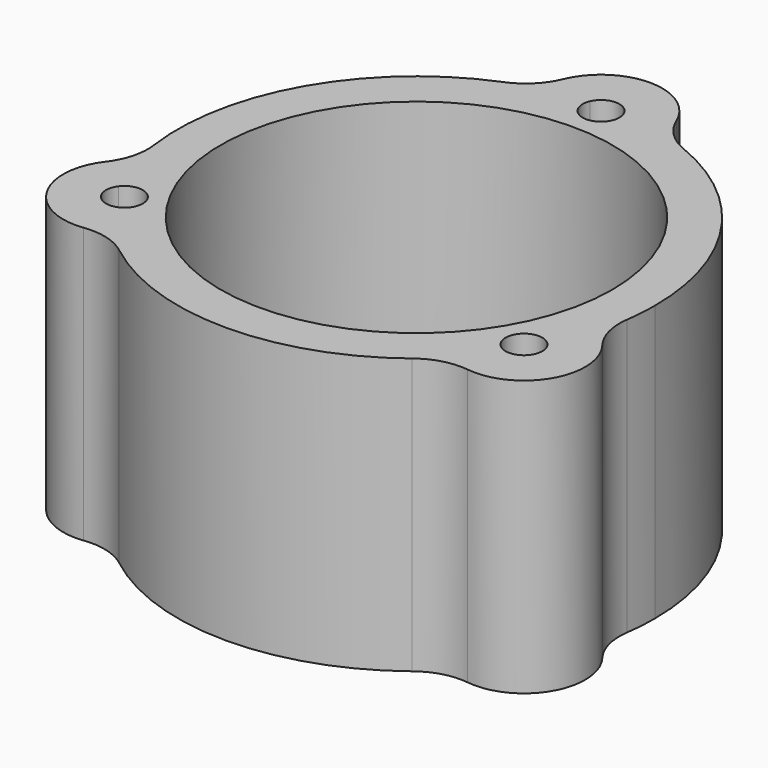
from build123d import *

# Parameters (mm, degrees)
F0_R     = 20.32
F1_DEPTH = 28.575
F2_R     = 6.35


with BuildPart() as f1:
    # F0 (on Top) → F1 (new body)
    with BuildSketch(Plane.XY):
        with BuildLine():
            ThreePointArc((23.9050999455, -6.4692674698), (24.5490837421, -3.2630832697), (24.765, 0))
            ThreePointArc((24.765, 0), (19.6285885254, 15.1004548773), (6.35, 23.9370575677))
            ThreePointArc((6.35, 23.9370575677), (4.0651088886, 24.4290833787), (1.7440091422, 24.703515076))
            ThreePointArc((1.7440091422, 24.703515076), (1.8643178935, 24.3286489263), (1.905, 23.9370575677))
            ThreePointArc((1.905, 23.9370575677), (-0.3915913586, 22.0727396742), (-1.7440091422, 24.703515076))
            ThreePointArc((-1.7440091422, 24.703515076), (-4.0651088886, 24.4290833787), (-6.35, 23.9370575677))
            ThreePointArc((-6.35, 23.9370575677), (-21.4471191247, 12.3825), (-23.9050999455, -6.4692674698))
            ThreePointArc((-23.9050999455, -6.4692674698), (-23.1887612414, -8.6940541227), (-22.2658761897, -10.8414013165))
            ThreePointArc((-22.2658761897, -10.8414013165), (-20.1370690632, -10.1581864481), (-18.8250999455, -11.9685287839))
            ThreePointArc((-18.8250999455, -11.9685287839), (-19.3113489683, -13.239815795), (-20.5218670475, -13.8621137596))
            ThreePointArc((-20.5218670475, -13.8621137596), (-19.1236523528, -15.735029256), (-17.5550999455, -17.4677900979))
            ThreePointArc((-17.5550999455, -17.4677900979), (0, -24.765), (17.5550999455, -17.4677900979))
            ThreePointArc((17.5550999455, -17.4677900979), (19.1236523528, -15.735029256), (20.5218670475, -13.8621137596))
            ThreePointArc((20.5218670475, -13.8621137596), (19.0803215513, -11.0160287839), (22.2658761897, -10.8414013165))
            ThreePointArc((22.2658761897, -10.8414013165), (23.1887612414, -8.6940541227), (23.9050999455, -6.4692674698))
        make_face()
        Circle(F0_R, mode=Mode.SUBTRACT)
        with BuildLine():
            ThreePointArc((-22.2658761897, -10.8414013165), (-23.1887612414, -8.6940541227), (-23.9050999455, -6.4692674698))
            ThreePointArc((-23.9050999455, -6.4692674698), (-26.2293612595, -15.1435287839), (-17.5550999455, -17.4677900979))
            ThreePointArc((-17.5550999455, -17.4677900979), (-19.1236523528, -15.735029256), (-20.5218670475, -13.8621137596))
            ThreePointArc((-20.5218670475, -13.8621137596), (-22.3798783397, -12.9210287839), (-22.2658761897, -10.8414013165))
        make_face()
        with BuildLine():
            ThreePointArc((1.7440091422, 24.703515076), (4.0651088886, 24.4290833787), (6.35, 23.9370575677))
            ThreePointArc((6.35, 23.9370575677), (0, 30.2870575677), (-6.35, 23.9370575677))
            ThreePointArc((-6.35, 23.9370575677), (-4.0651088886, 24.4290833787), (-1.7440091422, 24.703515076))
            ThreePointArc((-1.7440091422, 24.703515076), (0, 25.8420575677), (1.7440091422, 24.703515076))
        make_face()
        with BuildLine():
            ThreePointArc((17.5550999455, -17.4677900979), (26.2293612595, -15.1435287839), (23.9050999455, -6.4692674698))
            ThreePointArc((23.9050999455, -6.4692674698), (23.1887612414, -8.6940541227), (22.2658761897, -10.8414013165))
            ThreePointArc((22.2658761897, -10.8414013165), (22.5404422812, -11.3754979015), (22.6350999455, -11.9685287839))
            ThreePointArc((22.6350999455, -11.9685287839), (22.0013869566, -13.3872797611), (20.5218670475, -13.8621137596))
            ThreePointArc((20.5218670475, -13.8621137596), (19.1236523528, -15.735029256), (17.5550999455, -17.4677900979))
        make_face()
    extrude(amount=F1_DEPTH)

    # F2
    f2_edges = [f1.edges().sort_by_distance(p)[0] for p in [
        (6.35, 23.937058, 14.2875),
        (-23.9051, -6.469267, 14.2875),
        (17.5551, -17.46779, 14.2875),
        (23.9051, -6.469267, 14.2875),
        (-6.35, 23.937058, 14.2875),
        (-17.5551, -17.46779, 14.2875),
    ]]
    fillet(f2_edges, radius=F2_R)


solid = f1.part
